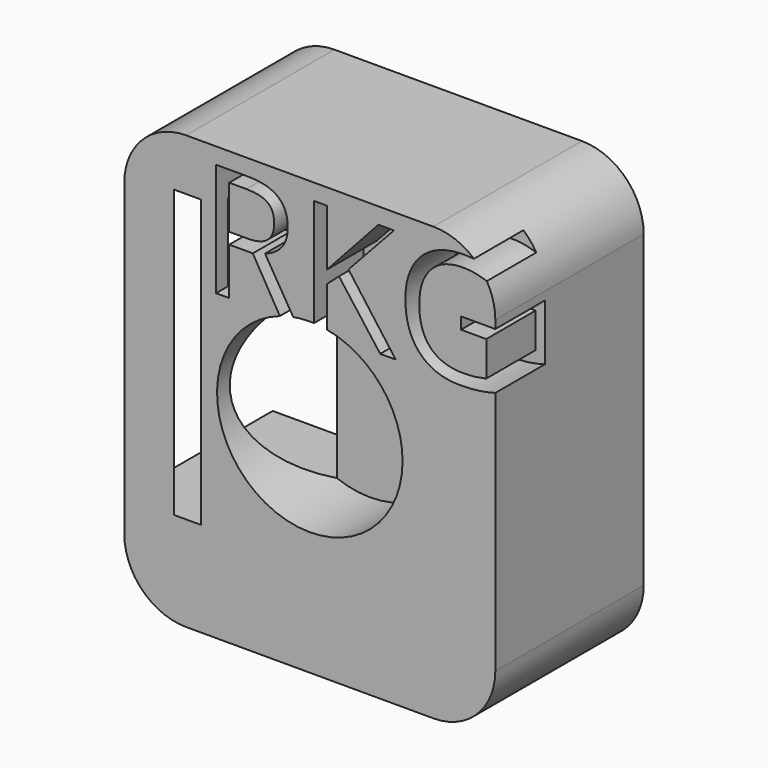
from build123d import *

# Parameters (mm, degrees)
F1_DEPTH     = 76.2
F2_R         = 38.1
F3_DEPTH     = 30.988
F4_R         = 38.1
F5_DEPTH     = 25.4
F7_W         = 91.167230159
F7_H         = 117.6627147943
F8_DEPTH     = 76.2
F9_TEXT_SIZE = 65.0760608487
F10_DEPTH    = 25.4


# Not quite as in the source:
# - Text() gives the source's letters only with a copy of the font that has no kerning and outlines rounded to 1/6400 em; it was checked with that copy


with BuildPart() as f1:
    # F0 (on Front) → F1 (new body)
    with BuildSketch(Plane.XZ):
        with BuildLine():
            Line((10.211761713, 121.2550016555), (-91.388238287, 121.2550016555))
            ThreePointArc((-91.388238287, 121.2550016555), (-109.3487505291, 113.8155138976), (-116.788238287, 95.8550016555))
            Line((-116.788238287, 95.8550016555), (-116.788238287, -31.1449983445))
            ThreePointArc((-116.788238287, -31.1449983445), (-109.3487505291, -49.1055105867), (-91.388238287, -56.5449983445))
            Line((-91.388238287, -56.5449983445), (10.211761713, -56.5449983445))
            ThreePointArc((10.211761713, -56.5449983445), (28.1722739552, -49.1055105867), (35.611761713, -31.1449983445))
            Line((35.611761713, -31.1449983445), (35.611761713, 95.8550016555))
            ThreePointArc((35.611761713, 95.8550016555), (28.1722739552, 113.8155138976), (10.211761713, 121.2550016555))
        make_face()
    extrude(amount=F1_DEPTH)

    # F2 (on face) → F3 (cut)
    with BuildSketch(Plane.XZ.offset(76.2)):
        with Locations((-40.588238287, 32.3550016555)):
            Circle(F2_R)
    extrude(amount=-F3_DEPTH, mode=Mode.SUBTRACT)

    # F4 (on face) → F5 (join)
    with BuildSketch(Plane(origin=(0, 0, 0), x_dir=(-1, 0, 0), z_dir=(0, 1, 0))):
        with Locations((40.588238287, 32.3550016555)):
            Circle(F4_R)
    extrude(amount=F5_DEPTH)

    # F7 (on face) → F8 (cut)
    with BuildSketch(Plane(origin=(-58.3941191435, 58.3941191435, 0), x_dir=(-0.7071067812, -0.7071067812, 0), z_dir=(-0.7071067812, 0.7071067812, 0))):
        with Locations((76.4564629644, 41.1868309602)):
            Rectangle(F7_W, F7_H)
    extrude(amount=-F8_DEPTH, mode=Mode.SUBTRACT)

    # F9 (on face) → F10 (cut)
    with BuildSketch(Plane.XZ.offset(76.2)):
        with Locations((-85.4767339381, 68.1584714512)):
            Text('RKG', F9_TEXT_SIZE, font='Open Sans', text_align=(TextAlign.LEFT, TextAlign.BOTTOM))
    extrude(amount=-F10_DEPTH, mode=Mode.SUBTRACT)


solid = f1.part
